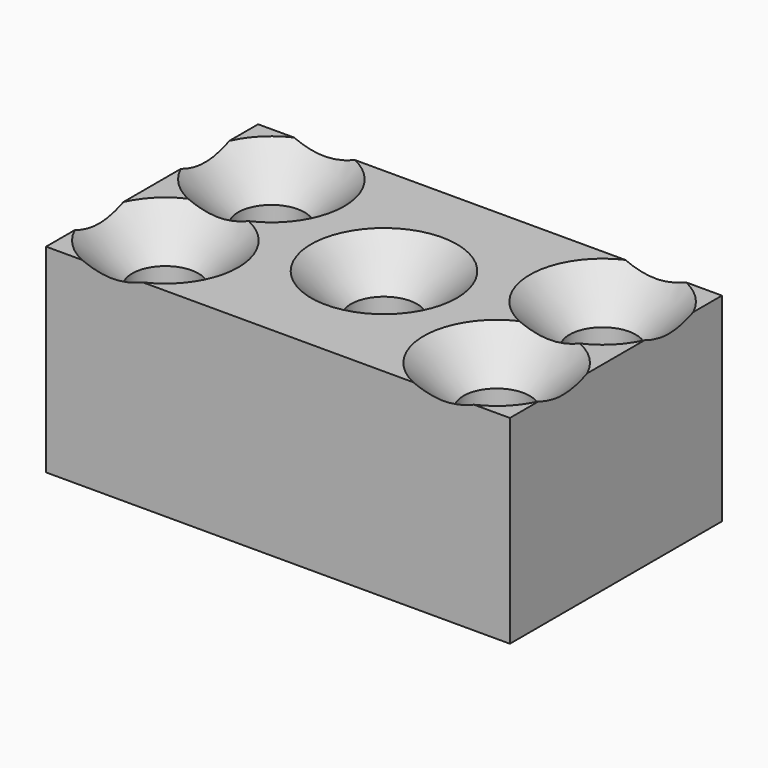
from build123d import *

# Parameters (mm, degrees)
F0_R     = 2.5
F1_DEPTH = 15


# Not quite as in the source:
# - a fillet or chamfer that OpenCascade refuses, or shapes differently, is made with other operations: its cross-section is extruded or revolved along the edge and cut away or added


with BuildPart() as f1:
    # F0 (on Top) → F1 (new body)
    with BuildSketch(Plane.XY):
        Polygon((-7.5, 10), (-17.5, 10), (-17.5, 5), (-17.5, -10), (17.5, -10), (17.5, 10), align=None)
        with Locations((-12.5, -5)):
            Circle(F0_R, mode=Mode.SUBTRACT)
        with Locations((12.5, -5)):
            Circle(F0_R, mode=Mode.SUBTRACT)
        with BuildLine():
            ThreePointArc((-10, 5), (-12.5, 2.5), (-15, 5))
            ThreePointArc((-15, 5), (-12.5, 7.5), (-10, 5))
        make_face(mode=Mode.SUBTRACT)
        Circle(F0_R, mode=Mode.SUBTRACT)
        with Locations((12.5, 5)):
            Circle(F0_R, mode=Mode.SUBTRACT)
    extrude(amount=F1_DEPTH)

    # F2: chamfer of 3 on 5 edges, made by hand

    # F2_s1 → F2_t2 (revolve, cut)
    with BuildSketch(Plane.XZ.offset(-5)):
        Polygon((-7, 15), (-10, 12), (-10, 15), align=None)
    revolve(axis=Axis((-12.5, 5, 15), (0, 0, 1)), mode=Mode.SUBTRACT)

    # F2_s3 → F2_t4 (revolve, cut)
    with BuildSketch(Plane.XZ):
        Polygon((5.5, 15), (2.5, 12), (2.5, 15), align=None)
    revolve(axis=Axis((0, 0, 15), (0, 0, 1)), mode=Mode.SUBTRACT)

    # F2_s5 → F2_t6 (revolve, cut)
    with BuildSketch(Plane.XZ.offset(5)):
        Polygon((-7, 15), (-10, 12), (-10, 15), align=None)
    revolve(axis=Axis((-12.5, -5, 15), (0, 0, 1)), mode=Mode.SUBTRACT)

    # F2_s7 → F2_t8 (revolve, cut)
    with BuildSketch(Plane.XZ.offset(-5)):
        Polygon((18, 15), (15, 12), (15, 15), align=None)
    revolve(axis=Axis((12.5, 5, 15), (0, 0, 1)), mode=Mode.SUBTRACT)

    # F2_s9 → F2_t10 (revolve, cut)
    with BuildSketch(Plane.XZ.offset(5)):
        Polygon((18, 15), (15, 12), (15, 15), align=None)
    revolve(axis=Axis((12.5, -5, 15), (0, 0, 1)), mode=Mode.SUBTRACT)


solid = f1.part
